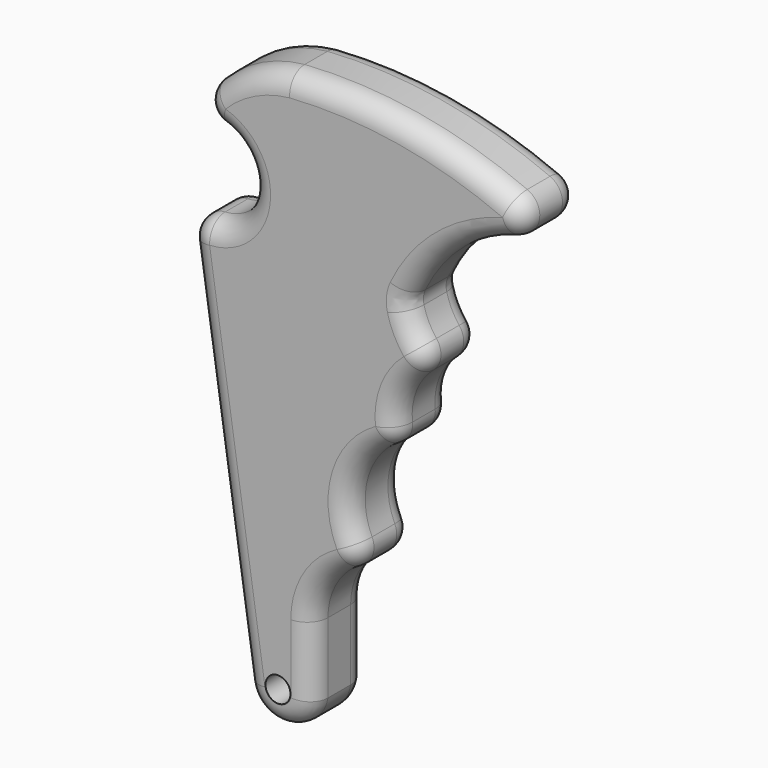
from build123d import *

# Parameters (mm, degrees)
F0_R     = 2.4195470085
F1_DEPTH = 13.5
F2_F1_R  = 4
F2_F2_R  = 4


with BuildPart() as f1:
    # F0 (on Front) → F1 (new body)
    with BuildSketch(Plane.XZ):
        with BuildLine():
            Line((-49.3356961767, 35.3497361023), (-37.7547828112, -42.2348335668))
            ThreePointArc((-37.7547828112, -42.2348335668), (-31.2758758664, -47.8184260428), (-24.7969689216, -42.2348335668))
            Line((-24.7969689216, -42.2348335668), (-24.7969689216, -28.5535179778))
            ThreePointArc((-24.7969689216, -28.5535179778), (-21.5958448136, -20.0642473306), (-13.5864750371, -15.8022164227))
            ThreePointArc((-13.5864750371, -15.8022164227), (-17.1539367925, -2.5764868036), (-7.7963641737, 7.4276394461))
            ThreePointArc((-7.7963641737, 7.4276394461), (-7.171857042, 16.766091593), (0, 22.7795069476))
            ThreePointArc((0, 22.7795069476), (-4.3611353912, 26.8073603633), (-6.4391756912, 32.3683722811))
            ThreePointArc((-6.4391756912, 32.3683722811), (7.334028543, 47.2529836996), (27.4388096167, 49.9082783979))
            ThreePointArc((27.4388096167, 49.9082783979), (0.2448615743, 61.737698638), (-29.2898025364, 64.4115739572))
            ThreePointArc((-29.2898025364, 64.4115739572), (-41.2715843547, 59.8673520775), (-49.3356961767, 49.9082783979))
            ThreePointArc((-49.3356961767, 49.9082783979), (-36.7089619026, 42.6290072501), (-49.3356961767, 35.3497361023))
        make_face()
        with Locations((-31.2758758664, -41.2677384298)):
            Circle(F0_R, mode=Mode.SUBTRACT)
    extrude(amount=F1_DEPTH)

    # F2: fillet of radius 4 on 26 edges, made by hand

    # F2_f1
    f2_f1_edges = [f1.edges().sort_by_distance(p)[0] for p in [
        (-6.4391756912, -6.75, 32.3683722811),
    ]]
    fillet(f2_f1_edges, radius=F2_F1_R)

    # F2_f2
    f2_f2_edges = [f1.edges().sort_by_distance(p)[0] for p in [
        (0, -6.75, 22.7795069476),
        (-3.9287601455, 0, 26.2022043612),
        (-3.9287601455, -13.5, 26.2022043612),
        (-7.7963641737, -6.75, 7.4276394461),
        (-7.171857042, 0, 16.766091593),
        (-7.171857042, -13.5, 16.766091593),
        (-13.5864750371, -6.75, -15.8022164227),
        (-17.1539367925, 0, -2.5764868036),
        (-17.1539367925, -13.5, -2.5764868036),
        (-21.5958448136, 0, -20.0642473306),
        (-21.5958448136, -13.5, -20.0642473306),
        (-49.3356961767, -6.75, 35.3497361023),
        (-43.545239494, 0, -3.4425487322),
        (-43.545239494, -13.5, -3.4425487322),
        (27.4388096167, -6.75, 49.9082783979),
        (-29.2898025364, -6.75, 64.4115739572),
        (0.2448615743, 0, 61.737698638),
        (0.2448615743, -13.5, 61.737698638),
        (-49.3356961767, -6.75, 49.9082783979),
        (-41.2715843547, 0, 59.8673520775),
        (-41.2715843547, -13.5, 59.8673520775),
        (-36.7089619026, 0, 42.6290072501),
        (-36.7089619026, -13.5, 42.6290072501),
        (-31.2758758664, -13.5, -47.8184260428),
        (-31.2758758664, 0, -47.8184260428),
        (-24.7969689216, -13.5, -35.3941757723),
        (-24.7969689216, 0, -35.3941757723),
        (-6.2638737515, -13.5, 32.2652253516),
        (-6.2638737515, 0, 32.2652253516),
    ]]
    fillet(f2_f2_edges, radius=F2_F2_R)


solid = f1.part
